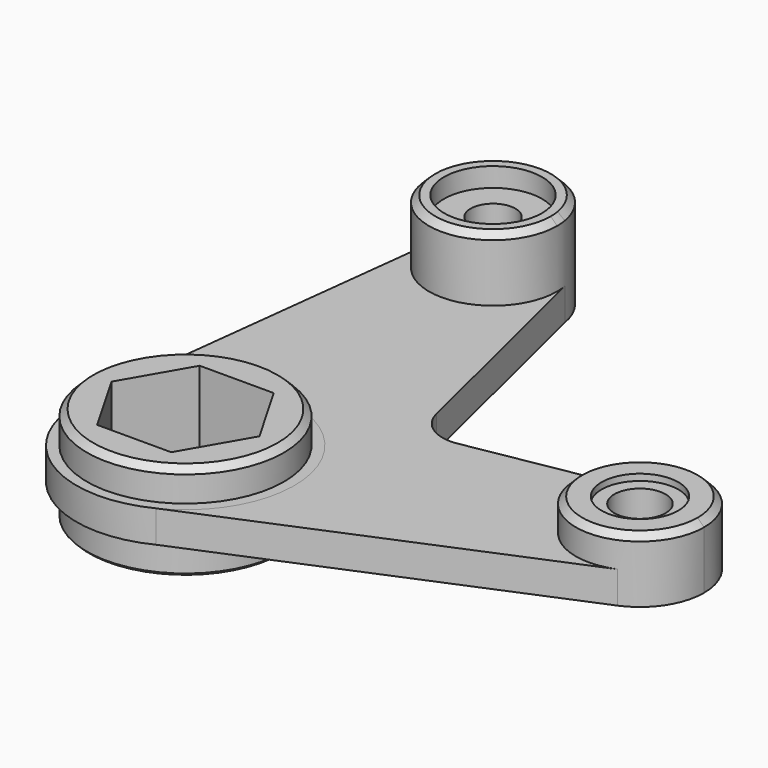
from build123d import *
from build123d import SkipClean  # not in build123d's __all__

# Parameters (mm, degrees)
F1_DEPTH  = 6.35
F0_R      = 19.5237916893
F2_DEPTH  = 12.7
F3_DEPTH  = 6.35
F4_DEPTH  = 12.7
F5_SIZE   = 1.27
F5_2_SIZE = 1.27
F6_R      = 4.445
F7_DEPTH  = 25.4
F8_R      = 9.7090709229
F9_DEPTH  = 3.81
F10_R     = 5.08
F11_DEPTH = 25.4
F10_R_2   = 7.62
F12_DEPTH = 1.27
F13_DEPTH = 6.35
F14_DEPTH = 6.35
F15_R     = 7.62
F16_SIZE  = 0.508


# Not quite as in the source:
# - after a boolean that leaves OpenCascade's solid faulty, fix() repairs it
# - a feature names something its author has since deleted; it is built from what else it names


with BuildPart() as f1:
    # F0 (on Top) → F1 (new body)
    with BuildSketch(Plane.XY):
        with BuildLine():
            ThreePointArc((12.5223688742, 78.3166666667), (12.6555143061, 77.2620535056), (12.7, 76.2))
            ThreePointArc((12.7, 76.2), (-0.7421013455, 63.5217002089), (-12.6132733217, 77.6816666667))
            Line((-12.6132733217, 77.6816666667), (-21.442564647, 2.5188333333))
            ThreePointArc((-21.442564647, 2.5188333333), (1.2615722873, 21.5531096449), (21.59, 0))
            ThreePointArc((21.59, 0), (18.3622941649, -11.3558026137), (9.644260954, -19.3162193674))
            Line((9.644260954, -19.3162193674), (78.13398925, 9.348603097))
            ThreePointArc((78.13398925, 9.348603097), (61.0445484479, 17.4882981523), (71.0267201121, 33.5712043384))
            Line((71.0267201121, 33.5712043384), (25.4411503373, 25.5379192568))
            Line((25.4411503373, 25.5379192568), (12.5223688742, 78.3166666667))
        make_face()
    extrude(amount=F1_DEPTH)

    # F0 (on Top) → F2, piece 2 (join)
    with BuildSketch(Plane.XY):
        with BuildLine():
            ThreePointArc((-12.6132733217, 77.6816666667), (-0.7421013455, 63.5217002089), (12.7, 76.2))
            ThreePointArc((12.7, 76.2), (12.6555143061, 77.2620535056), (12.5223688742, 78.3166666667))
            ThreePointArc((12.5223688742, 78.3166666667), (-0.3207368932, 88.8959492692), (-12.6132733217, 77.6816666667))
        make_face()
    extrude(amount=F2_DEPTH)

    # F3 (add): a face of the model
    f3_faces = [f1.faces().sort_by_distance(p)[0] for p in [
        (0, 76.2, 12.7),
    ]]
    with SkipClean():  # cleaning this boolean's faces spoils the solid; the shape is the same uncleaned
        extrude(f3_faces, amount=F3_DEPTH)

    # F0 (on Top) → F4 (join)
    with BuildSketch(Plane.XY):
        with BuildLine():
            ThreePointArc((85.9308064152, 21.0639263144), (81.3946934781, 30.792284245), (71.0267201121, 33.5712043384))
            ThreePointArc((71.0267201121, 33.5712043384), (61.0445484479, 17.4882981523), (78.13398925, 9.348603097))
            ThreePointArc((78.13398925, 9.348603097), (83.8034225059, 14.0276070352), (85.9308064152, 21.0639263144))
        make_face()
    extrude(amount=F4_DEPTH)

    add(f1.part.fix(), mode=Mode.REPLACE)

    # F5
    f5_edges = [f1.edges().sort_by_distance(p)[0] for p in [
        (-12.7, 76.2, 19.05),
        (68.327624, 32.77925, 12.7),
    ]]
    chamfer(f5_edges, length=F5_SIZE)

    # F6 (on face) → F7 (cut)
    with BuildSketch(Plane.XY.offset(19.05)):
        with Locations((0, 76.2)):
            Circle(F6_R)
    extrude(amount=-F7_DEPTH, mode=Mode.SUBTRACT)

    # F8 (on face) → F9 (cut)
    with BuildSketch(Plane.XY.offset(19.05)):
        with Locations((0, 76.2)):
            Circle(F8_R)
    extrude(amount=-F9_DEPTH, mode=Mode.SUBTRACT)

    # F10 (on face) → F11 (cut)
    with BuildSketch(Plane.XY.offset(12.7)):
        with Locations((73.2308064152, 21.0639263144)):
            Circle(F10_R)
    extrude(amount=-F11_DEPTH, mode=Mode.SUBTRACT)

    # F10 (on face) → F12 (cut)
    with BuildSketch(Plane.XY.offset(12.7)):
        with Locations((73.2308064152, 21.0639263144)):
            Circle(F10_R_2)
        with Locations((73.2308064152, 21.0639263144)):
            Circle(F10_R, mode=Mode.SUBTRACT)
    extrude(amount=-F12_DEPTH, mode=Mode.SUBTRACT)

    # F15
    f15_edges = [f1.edges().sort_by_distance(p)[0] for p in [
        (25.44115, 25.537919, 3.175),
    ]]
    fillet(f15_edges, radius=F15_R)


with BuildPart() as f2:
    # F0 (on Top) → F2 (new body)
    with BuildSketch(Plane.XY):
        Circle(F0_R)
        Polygon((-14.6646968374, 0), (-7.3323484187, 12.7), (7.3323484187, 12.7), (14.6646968374, 0), (7.3323484187, -12.7), (-7.3323484187, -12.7), align=None, mode=Mode.SUBTRACT)
    extrude(amount=F2_DEPTH)

    # F5#2
    f5_2_edges = [f2.edges().sort_by_distance(p)[0] for p in [
        (-19.523792, 0, 12.7),
    ]]
    chamfer(f5_2_edges, length=F5_2_SIZE)

    # F14 (add): a face of the model
    f14_faces = [f2.faces().sort_by_distance(p)[0] for p in [
        (-18.9715754694, 0, 0),
    ]]
    extrude(f14_faces, amount=F14_DEPTH)

    # F16
    f16_edges = [f2.edges().sort_by_distance(p)[0] for p in [
        (-19.523792, 0, -6.35),
    ]]
    chamfer(f16_edges, length=F16_SIZE)


with BuildPart() as f13:
    # F0 (on Top) → F13 (new body)
    with BuildSketch(Plane.XY):
        with BuildLine():
            ThreePointArc((21.59, 0), (1.2615722873, 21.5531096449), (-21.442564647, 2.5188333333))
            ThreePointArc((-21.442564647, 2.5188333333), (-12.4093663867, -17.6673632974), (9.644260954, -19.3162193674))
            ThreePointArc((9.644260954, -19.3162193674), (18.3622941649, -11.3558026137), (21.59, 0))
        make_face()
        Circle(F0_R, mode=Mode.SUBTRACT)
    extrude(amount=F13_DEPTH)


solid = Compound([f1.part, f2.part, f13.part])
